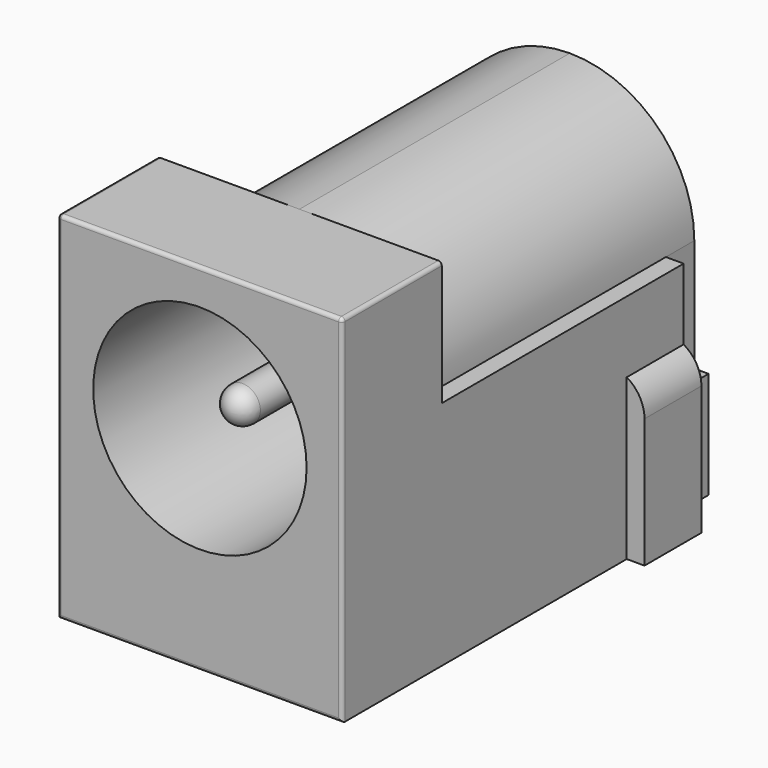
from build123d import *

# Parameters (mm, degrees)
F0_W         = 8
F0_H         = 10
F0_R         = 3
F1_DEPTH     = 12
F2_W         = 1
F2_H         = 10
F3_DEPTH     = 8
F5_DEPTH     = 9.5
F4_W         = 0.5
F4_H         = 6.5
F6_DEPTH     = 1
F7_R         = 0.5
F8_DEPTH     = 11
F9_R         = 0.5
F10_R        = 0.1
F11_W        = 2
F11_H        = 3
F12_DEPTH    = 0.5
F13_R        = 0.375
F14_DEPTH    = 0.25
F15_W        = 2
F15_H        = 4.5
F16_DEPTH    = 0.5
F17_T1_DEPTH = 6.3301270189


# Not quite as in the source:
# - a fillet or chamfer that OpenCascade refuses, or shapes differently, is made with other operations: its cross-section is extruded or revolved along the edge and cut away or added


with BuildPart() as f1:
    # F0 (on Front) → F1 (new body)
    with BuildSketch(Plane.XZ):
        with Locations((-29.9816446145, 7.3587873485)):
            Rectangle(F0_W, F0_H)
        with Locations((-29.9816446145, 8.3587873485)):
            Circle(F0_R, mode=Mode.SUBTRACT)
    extrude(amount=F1_DEPTH)

    # F2 (on face) → F3 (join, through all)
    with BuildSketch(Plane(origin=(-33.9816446145, 0, 0), x_dir=(0, -1, 0), z_dir=(-1, 0, 0))):
        with Locations((-0.5, 7.3587873485)):
            Rectangle(F2_W, F2_H)
    extrude(amount=-F3_DEPTH)

    # F4 (on face) → F5 (cut)
    with BuildSketch(Plane(origin=(0, 1, 0), x_dir=(-1, 0, 0), z_dir=(0, 1, 0))):
        with BuildLine():
            Line((33.9816446145, 12.3587873485), (29.9816446145, 12.3587873485))
            ThreePointArc((29.9816446145, 12.3587873485), (32.4565183487, 11.3336610826), (33.4816446145, 8.8587873485))
            Line((33.4816446145, 8.8587873485), (33.9816446145, 8.8587873485))
            Line((33.9816446145, 8.8587873485), (33.9816446145, 12.3587873485))
        make_face()
        with BuildLine():
            Line((29.9816446145, 12.3587873485), (25.9816446145, 12.3587873485))
            Line((25.9816446145, 12.3587873485), (25.9816446145, 8.8587873485))
            Line((25.9816446145, 8.8587873485), (26.4816446145, 8.8587873485))
            ThreePointArc((26.4816446145, 8.8587873485), (27.5067708804, 11.3336610826), (29.9816446145, 12.3587873485))
        make_face()
    extrude(amount=-F5_DEPTH, mode=Mode.SUBTRACT)

    # F4 (on face) → F6 (cut)
    with BuildSketch(Plane(origin=(0, 1, 0), x_dir=(-1, 0, 0), z_dir=(0, 1, 0))):
        with Locations((26.2316446145, 5.6087873485)):
            Rectangle(F4_W, F4_H)
        with Locations((33.7316446145, 5.6087873485)):
            Rectangle(F4_W, F4_H)
    extrude(amount=-F6_DEPTH, mode=Mode.SUBTRACT)

    # F7 (on face) → F8 (join)
    with BuildSketch(Plane.XZ):
        with Locations((-29.9816446145, 8.3587873485)):
            Circle(F7_R)
    extrude(amount=F8_DEPTH)

    # F9
    f9_edges = [f1.edges().sort_by_distance(p)[0] for p in [
        (-30.481645, -11, 8.358787),
    ]]
    fillet(f9_edges, radius=F9_R)

    # F10
    f10_edges = [f1.edges().sort_by_distance(p)[0] for p in [
        (-29.981645, -12, 12.358787),
        (-25.981645, -12, 7.358787),
        (-33.981645, -12, 7.358787),
        (-29.981645, -12, 2.358787),
        (-25.981645, -10.25, 12.358787),
        (-33.981645, -10.25, 12.358787),
    ]]
    fillet(f10_edges, radius=F10_R)

    # F11 (on face) → F12 (join)
    with BuildSketch(Plane(origin=(0, 1, 0), x_dir=(-1, 0, 0), z_dir=(0, 1, 0))):
        with Locations((27.4816446145, 3.8587873485)):
            Rectangle(F11_W, F11_H)
        with Locations((32.4816446145, 3.8587873485)):
            Rectangle(F11_W, F11_H)
    extrude(amount=F12_DEPTH)

    # F13 (on face) → F14 (join)
    with BuildSketch(Plane(origin=(0, 1, 0), x_dir=(-1, 0, 0), z_dir=(0, 1, 0))):
        with BuildLine():
            Line((31.4816446145, 6.8587873485), (28.4816446145, 6.8587873485))
            ThreePointArc((28.4816446145, 6.8587873485), (29.9816446145, 6.3587873485), (31.4816446145, 6.8587873485))
        make_face()
        with BuildLine():
            ThreePointArc((31.4816446145, 6.8587873485), (32.217712592, 7.7407533597), (32.4816446145, 8.8587873485))
            ThreePointArc((32.4816446145, 8.8587873485), (28.8636106257, 11.094855326), (28.4816446145, 6.8587873485))
            Line((28.4816446145, 6.8587873485), (31.4816446145, 6.8587873485))
        make_face()
        with BuildLine():
            ThreePointArc((31.4816446145, 6.8587873485), (29.9816446145, 6.3587873485), (28.4816446145, 6.8587873485))
            Line((28.4816446145, 6.8587873485), (28.4816446145, 5.3587873485))
            Line((28.4816446145, 5.3587873485), (28.4816446145, 2.3587873485))
            Line((28.4816446145, 2.3587873485), (31.4816446145, 2.3587873485))
            Line((31.4816446145, 2.3587873485), (31.4816446145, 5.3587873485))
            Line((31.4816446145, 5.3587873485), (31.4816446145, 6.8587873485))
        make_face()
        with Locations((29.9816446145, 4.8587873485)):
            Circle(F13_R, mode=Mode.SUBTRACT)
    extrude(amount=F14_DEPTH)

    # F15 (on face) → F16 (join)
    with BuildSketch(Plane.YZ.offset(-25.9816446145)):
        with Locations((-1, 4.6087873485)):
            Rectangle(F15_W, F15_H)
    extrude(amount=F16_DEPTH)

    # F17: fillet of radius 1 on 1 edges, made by hand

    # F17_s2 → F17_t1 (cut)
    with BuildSketch(Plane.XZ.offset(-2.1650635095)):
        with BuildLine():
            ThreePointArc((-25.9816446145, 6.8587873485), (-25.6156192107, 6.4927619447), (-25.4816446145, 5.9927619447))
            Line((-25.4816446145, 5.9927619447), (-25.4816446145, 6.8587873485))
            Line((-25.4816446145, 6.8587873485), (-25.9816446145, 6.8587873485))
        make_face()
    extrude(amount=F17_T1_DEPTH, mode=Mode.SUBTRACT)


solid = f1.part
